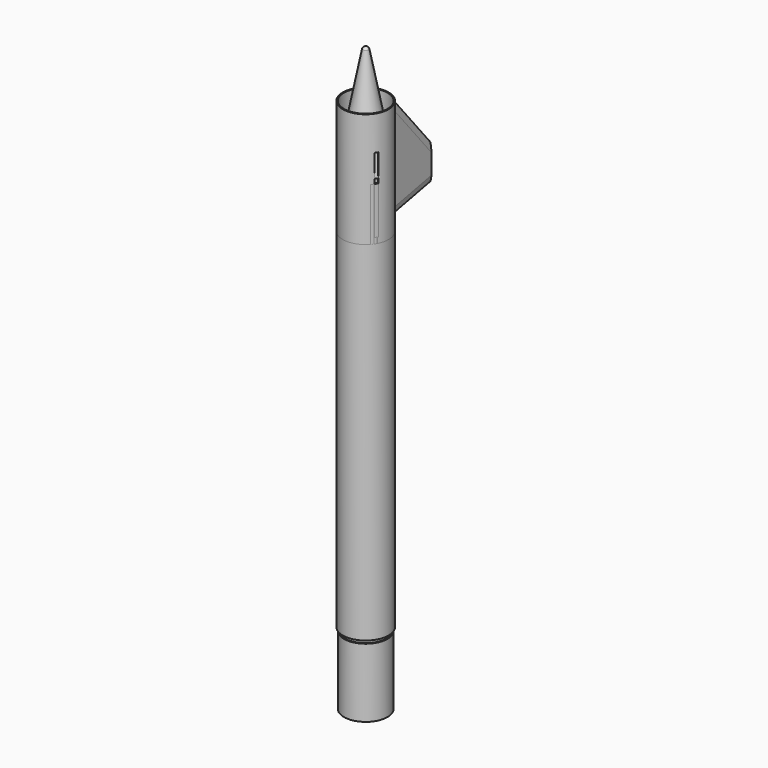
from build123d import *

# Parameters (mm, degrees)
F2_W         = 1
F2_H         = 350
F4_W         = 1
F4_H         = 60
F8_W         = 1
F8_H         = 100
F11_W        = 3
F11_H        = 5
F12_DEPTH    = 65
F14_DEPTH    = 1.5
F15_C1_SIZE2 = 5
F15_C1_SIZE  = 1
F15_C2_SIZE2 = 5
F15_C2_SIZE  = 1
F15_C3_SIZE2 = 1
F15_C3_SIZE  = 5
F15_C4_SIZE2 = 5
F15_C4_SIZE  = 1
F17_R        = 19
F17_R_2      = 9
F18_DEPTH    = 4
F19_R        = 19
F19_R_2      = 1
F19_R_3      = 8
F20_DEPTH    = 4


# Not quite as in the source:
# - two fillets or chamfers of one size are made in one step


with BuildPart() as f1:
    # F0 (on Front) → F1 (revolve)
    with BuildSketch(Plane.XZ):
        with BuildLine():
            Line((0, 91.6925824036), (0, -25))
            Line((0, -25), (19, -25))
            Line((19, -25), (19, 0))
            Line((19, 0), (20, 0))
            Line((20, 0), (2.5, 90))
            ThreePointArc((2.5, 90), (1.5095392669, 91.2296392537), (0, 91.6925824036))
        make_face()
    revolve(axis=Axis((0, 0, 33.3462912018), (0, 0, -1)))


with BuildPart() as f3:
    # F2 (on Front) → F3 (revolve)
    with BuildSketch(Plane.XZ):
        with Locations((19.5, -179)):
            Rectangle(F2_W, F2_H)
    revolve(axis=Axis((0, 0, -177), (0, 0, -1)))


with BuildPart() as f5:
    # F4 (on Front) → F5 (revolve)
    with BuildSketch(Plane.XZ):
        with Locations((18.5, -387)):
            Rectangle(F4_W, F4_H)
    revolve(axis=Axis((0, 0, -341.6038751602), (0, 0, -1)))


with BuildPart() as f7:
    # F6 (on Front) → F7 (revolve)
    with BuildSketch(Plane.XZ):
        Polygon((18, 0), (17, 0), (17, -30), (0.7, -30), (0.7, -34), (17, -34), (17, -50), (18, -50), align=None)
    revolve(axis=Axis((0, 0, -50), (0, 0, -1)))


with BuildPart() as f9:
    # F8 (on Front) → F9 (revolve)
    with BuildSketch(Plane.XZ):
        with Locations((19.5, 0)):
            Rectangle(F8_W, F8_H)
    revolve(axis=Axis((0, 0, 0), (0, 0, -1)))

    # F11 (on offset) → F12 (cut)
    with BuildSketch(Plane.XY.offset(20)):
        Polygon((-19.7582219053, -9.6753639281), (-18.2582219053, -12.2734401395), (-13.9280948863, -9.7734401395), (-15.4280948863, -7.1753639281), align=None)
        Polygon((18.2582219053, -12.2734401395), (19.7582219053, -9.6753639281), (15.4280948863, -7.1753639281), (13.9280948863, -9.7734401395), align=None)
        with Locations((0, 19.4488040676)):
            Rectangle(F11_W, F11_H)
    extrude(amount=-F12_DEPTH, mode=Mode.SUBTRACT)


with BuildPart() as f14:
    # F13 (on Right) → F14 (new body, symmetric)
    with BuildSketch(Plane.YZ):
        Polygon((70, -10), (20, 50), (20, 16), (15, 16), (15, -45), (20, -45), (20, -50), (70, -40), align=None)
    extrude(amount=F14_DEPTH, both=True)

    # F15: chamfer of 1 x 5 on 4 edges, made by hand

    # F15_c1
    f15_c1_edges = [f14.edges().sort_by_distance(p)[0] for p in [
        (-1.5, 45, 20),
    ]]
    f15_c1_side = f14.faces().sort_by_distance((-1.48, 45, 20))[0]
    chamfer(f15_c1_edges, length=F15_C1_SIZE, length2=F15_C1_SIZE2, reference=f15_c1_side)

    # F15_c2
    f15_c2_edges = [f14.edges().sort_by_distance(p)[0] for p in [
        (1.5, 45, 20),
    ]]
    f15_c2_side = f14.faces().sort_by_distance((1.48, 45, 20))[0]
    chamfer(f15_c2_edges, length=F15_C2_SIZE, length2=F15_C2_SIZE2, reference=f15_c2_side)

    # F15_c3
    f15_c3_edges = [f14.edges().sort_by_distance(p)[0] for p in [
        (-1.5, 45, -45),
    ]]
    f15_c3_side = f14.faces().sort_by_distance((-1.5, 44.9960776773, -44.9803883865))[0]
    chamfer(f15_c3_edges, length=F15_C3_SIZE, length2=F15_C3_SIZE2, reference=f15_c3_side)

    # F15_c4
    f15_c4_edges = [f14.edges().sort_by_distance(p)[0] for p in [
        (1.5, 45, -45),
    ]]
    f15_c4_side = f14.faces().sort_by_distance((1.48, 45, -45))[0]
    chamfer(f15_c4_edges, length=F15_C4_SIZE, length2=F15_C4_SIZE2, reference=f15_c4_side)


with BuildPart() as f18:
    # F17 (on Top) → F18 (new body)
    with BuildSketch(Plane.XY):
        Circle(F17_R)
        Circle(F17_R_2, mode=Mode.SUBTRACT)
    extrude(amount=F18_DEPTH)


with BuildPart() as f20:
    # F19 (on offset) → F20 (new body)
    with BuildSketch(Plane.XY.offset(20)):
        Circle(F19_R)
        with Locations((-10, 10)):
            Circle(F19_R_2, mode=Mode.SUBTRACT)
        Circle(F19_R_3, mode=Mode.SUBTRACT)
    extrude(amount=F20_DEPTH)


with BuildPart() as f22:
    # F21 (on Front) → F22 (revolve)
    with BuildSketch(Plane.XZ):
        Polygon((7, -32), (0, -32), (0, -73), (1.5, -73), (1.5, -93), (7, -98), (7, -100), (9, -100), (9, -30), (7, -30), align=None)
    revolve(axis=Axis((0, 0, -65), (0, 0, -1)))


solid = Compound([f1.part, f3.part, f5.part, f7.part, f9.part, f14.part, f18.part, f20.part, f22.part])
